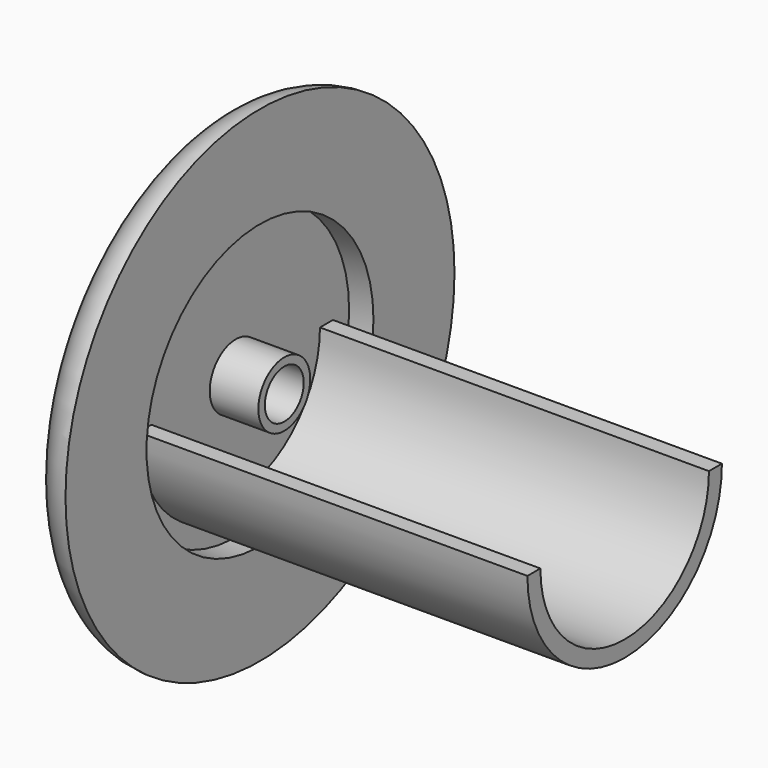
from build123d import *

# Parameters (mm, degrees)
F0_R     = 30
F1_DEPTH = 5
F2_R     = 4.99999
F3_R     = 17.5
F4_DEPTH = 3
F5_R     = 4
F5_R_2   = 3
F6_DEPTH = 6
F8_DEPTH = 50


# Not quite as in the source:
# - a fillet or chamfer is up to 0.001 mm smaller than in the source, because OpenCascade refuses the exact size


with BuildPart() as f1:
    # F0 (on Right) → F1 (new body)
    with BuildSketch(Plane.YZ):
        Circle(F0_R)
    extrude(amount=F1_DEPTH)

    # F2 (radius 5 in the source; OpenCascade refuses exactly that, so slightly less here)
    f2_edges = [f1.edges().sort_by_distance(p)[0] for p in [
        (0, -30, 0),
    ]]
    fillet(f2_edges, radius=F2_R)

    # F3 (on face) → F4 (cut)
    with BuildSketch(Plane.YZ.offset(5)):
        Circle(F3_R)
    extrude(amount=-F4_DEPTH, mode=Mode.SUBTRACT)

    # F5 (on face) → F6 (join)
    with BuildSketch(Plane.YZ.offset(2)):
        Circle(F5_R)
        Circle(F5_R_2, mode=Mode.SUBTRACT)
    extrude(amount=F6_DEPTH)


with BuildPart() as f8:
    # F7 (on Right) → F8 (new body)
    with BuildSketch(Plane.YZ):
        with BuildLine():
            Line((-13, 0), (-15, 0))
            ThreePointArc((-15, 0), (0, -15), (15, 0))
            Line((15, 0), (13, 0))
            ThreePointArc((13, 0), (0, -13), (-13, 0))
        make_face()
    extrude(amount=F8_DEPTH)


solid = Compound([f1.part, f8.part])
